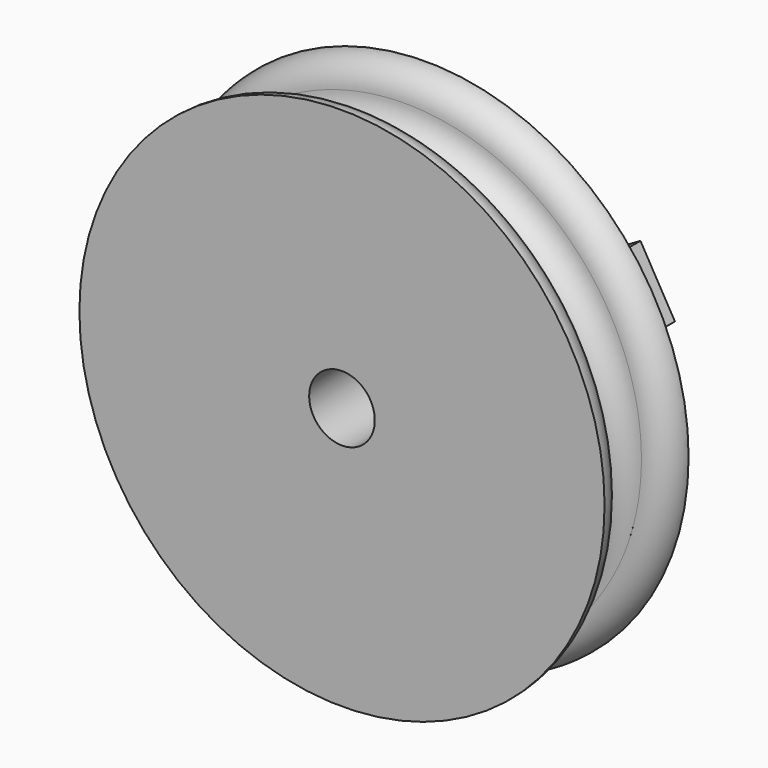
from build123d import *

# Parameters (mm, degrees)
F0_R      = 20.32
F1_DEPTH  = 2.54
F2_R      = 25.4
F3_DEPTH  = 2.54
F4_R      = 25.4
F5_DEPTH  = 2.54
F6_R      = 2.53999
F7_R      = 3.175
F8_DEPTH  = 25.4
F9_DEPTH  = 0.254
F11_DEPTH = 5.08
F10_W     = 6.6752280109
F10_H     = 6.1189569533


# Not quite as in the source:
# - a fillet or chamfer is up to 0.001 mm smaller than in the source, because OpenCascade refuses the exact size


with BuildPart() as f1:
    # F0 (on Front) → F1 (new body, symmetric)
    with BuildSketch(Plane.XZ):
        Circle(F0_R)
    extrude(amount=F1_DEPTH, both=True)

    # F2 (on face) → F3 (join)
    with BuildSketch(Plane.XZ.offset(2.54)):
        Circle(F2_R)
    extrude(amount=F3_DEPTH)

    # F4 (on face) → F5 (join)
    with BuildSketch(Plane(origin=(0, 2.54, 0), x_dir=(-1, 0, 0), z_dir=(0, 1, 0))):
        Circle(F4_R)
    extrude(amount=F5_DEPTH)

    # F6 (radius 2.54 in the source; OpenCascade refuses exactly that, so slightly less here)
    f6_edges = [f1.edges().sort_by_distance(p)[0] for p in [
        (-20.32, 2.54, 0),
        (20.32, 0, 0),
        (-20.32, -2.54, 0),
        (25.4, 2.54, 0),
        (-25.4, -2.54, 0),
    ]]
    fillet(f6_edges, radius=F6_R)

    # F7 (on face) → F8 (cut)
    with BuildSketch(Plane(origin=(0, 5.08, 0), x_dir=(-1, 0, 0), z_dir=(0, 1, 0))):
        Circle(F7_R)
    extrude(amount=-F8_DEPTH, mode=Mode.SUBTRACT)

    # F7 (on face) → F9 (join)
    with BuildSketch(Plane(origin=(0, 5.08, 0), x_dir=(-1, 0, 0), z_dir=(0, 1, 0))):
        with Locations((0, 18.4368621558)):
            Circle(F7_R)
    extrude(amount=F9_DEPTH)


with BuildPart() as f11:
    # F10 (on face) → F11 (new body)
    with BuildSketch(Plane(origin=(0, 5.08, 0), x_dir=(-1, 0, 0), z_dir=(0, 1, 0))):
        Polygon((20.0151837326, 7.7018270269), (16.6775697272, 13.4827440604), (11.378397561, 10.4232655838), (14.7160115664, 4.6423485503), align=None)
    extrude(amount=F11_DEPTH)


with BuildPart() as f11b:
    # F10 (on face) → F11, piece 2 (new body)
    with BuildSketch(Plane(origin=(0, 5.08, 0), x_dir=(-1, 0, 0), z_dir=(0, 1, 0))):
        with Locations((0, -18.1250926107)):
            Rectangle(F10_W, F10_H)
    extrude(amount=F11_DEPTH)


with BuildPart() as f11c:
    # F10 (on face) → F11, piece 3 (new body)
    with BuildSketch(Plane(origin=(0, 5.08, 0), x_dir=(-1, 0, 0), z_dir=(0, 1, 0))):
        Polygon((-16.6775697272, 13.4827440604), (-20.0151837326, 7.7018270269), (-14.7160115664, 4.6423485503), (-11.378397561, 10.4232655838), align=None)
    extrude(amount=F11_DEPTH)


solid = Compound([f1.part, f11.part, f11b.part, f11c.part])
